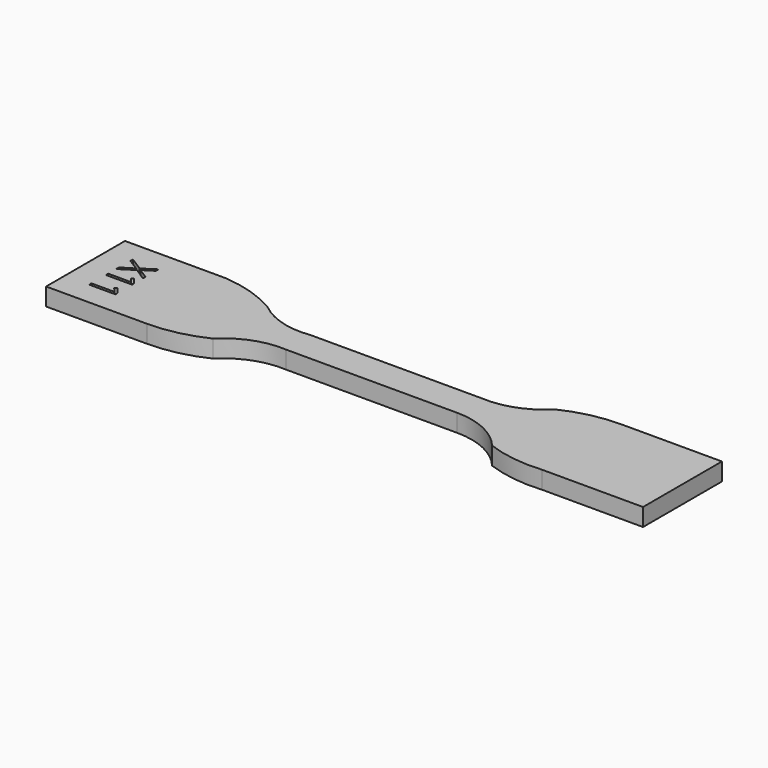
from build123d import *

# Parameters (mm, degrees)
F1_DEPTH     = 3.4
F2_TEXT_SIZE = 7.0564552314
F3_DEPTH     = 1


# Not quite as in the source:
# - Text() gives the source's letters only with a copy of the font that has no kerning and outlines rounded to 1/6400 em; it was checked with that copy


with BuildPart() as f1:
    # F0 (on Top) → F1 (new body)
    with BuildSketch(Plane.XY):
        with BuildLine():
            Line((-14.4320548165, 19.7811394548), (-33.8720548165, 19.7811394548))
            Line((-33.8720548165, 19.7811394548), (-33.8720548165, 0.7811394548))
            Line((-33.8720548165, 0.7811394548), (-14.4320548165, 0.7811394548))
            ThreePointArc((-14.4320548165, 0.7811394548), (-8.9053122052, 1.3996892086), (-3.6520548165, 3.2247301661))
            ThreePointArc((-3.6520548165, 3.2247301661), (1.3014698263, 6.4128780055), (7.1279451835, 7.2811394548))
            Line((7.1279451835, 7.2811394548), (40.1279451835, 7.2811394548))
            ThreePointArc((40.1279451835, 7.2811394548), (46.0837574042, 5.9511158081), (50.9079451835, 2.2137538538))
            ThreePointArc((50.9079451835, 2.2137538538), (56.2191047011, 0.9041953221), (61.6879451835, 0.7811394548))
            Line((61.6879451835, 0.7811394548), (81.1279451835, 0.7811394548))
            Line((81.1279451835, 0.7811394548), (81.1279451835, 19.7811394548))
            Line((81.1279451835, 19.7811394548), (61.6879451835, 19.7811394548))
            ThreePointArc((61.6879451835, 19.7811394548), (56.1612025723, 19.162589701), (50.9079451835, 17.3375487435))
            ThreePointArc((50.9079451835, 17.3375487435), (45.9544205407, 14.1494009041), (40.1279451835, 13.2811394548))
            Line((40.1279451835, 13.2811394548), (7.1279451835, 13.2811394548))
            ThreePointArc((7.1279451835, 13.2811394548), (1.4167452884, 13.6925537245), (-3.6520548165, 16.3560723447))
            ThreePointArc((-3.6520548165, 16.3560723447), (-8.8458057958, 18.686276846), (-14.4320548165, 19.7811394548))
        make_face()
    extrude(amount=F1_DEPTH)

    # F2 (on face) → F3 (cut)
    with BuildSketch(Plane.XY.offset(3.4)):
        with Locations(Location((-29.1824135929, 15.8650862949), (0, 0, -90))):
            Text('X11', F2_TEXT_SIZE, font='Open Sans', text_align=(TextAlign.LEFT, TextAlign.BOTTOM))
    extrude(amount=-F3_DEPTH, mode=Mode.SUBTRACT)


solid = f1.part
